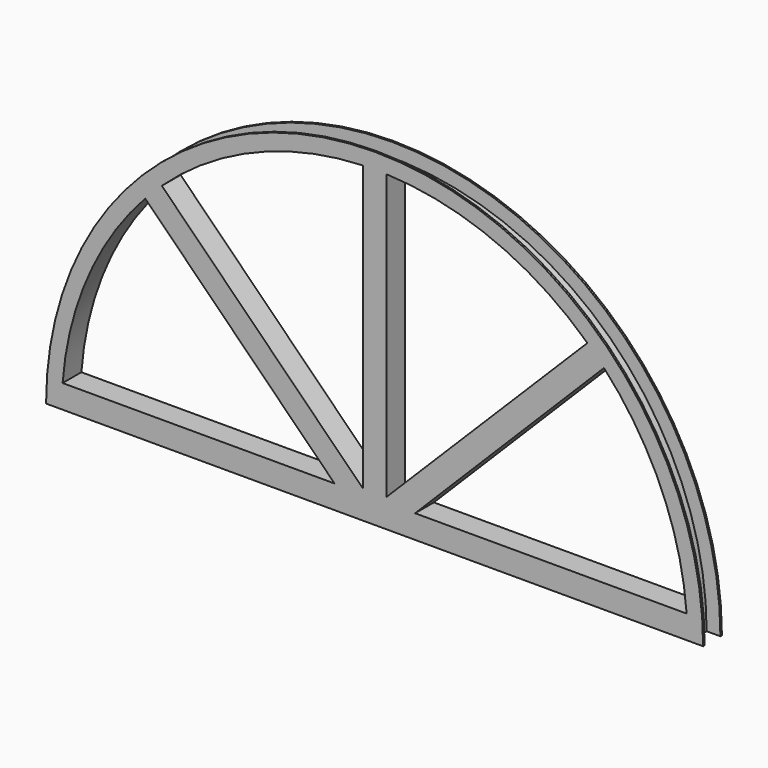
from build123d import *

# Parameters (mm, degrees)
F1_DEPTH     = 75
F2_T         = -6
F3_W         = 75
F3_H         = 75
F4_DEPTH     = 1000
F6_W         = 75
F6_H         = 75
F7_DEPTH     = 1000
F9_DEPTH     = 75
F11_DEPTH    = 75
F12_T        = 6
F12_T3_DEPTH = 87
F12_T6_ANGLE = 180.000000001
F12_T8_ANGLE = 180.000000001


# Not quite as in the source:
# - a shell that OpenCascade refuses in one call is made with other operations: the cavity is built on its own and cut out


with BuildPart() as f1:
    # F0 (on Front) → F1 (new body)
    with BuildSketch(Plane.XZ):
        with BuildLine():
            ThreePointArc((707.1067811865, 707.1067811865), (923.8795325113, 382.6834323651), (1000, 0))
            Line((1000, 0), (1050, 0))
            ThreePointArc((1050, 0), (0, 1050), (-1050, 0))
            Line((-1050, 0), (-1000, 0))
            ThreePointArc((-1000, 0), (-923.8795325113, 382.6834323651), (-707.1067811865, 707.1067811865))
            ThreePointArc((-707.1067811865, 707.1067811865), (-382.6834323651, 923.8795325113), (0, 1000))
            ThreePointArc((0, 1000), (382.6834323651, 923.8795325113), (707.1067811865, 707.1067811865))
        make_face()
    extrude(amount=F1_DEPTH)

    # F2
    f2_openings = [f1.faces().sort_by_distance(p)[0] for p in [
        (0, -37.5, 1050),
        (1025, -37.5, 0),
        (-1025, -37.5, 0),
    ]]
    offset(amount=F2_T, openings=f2_openings)

    # F3 (on Right) → F4 (join)
    with BuildSketch(Plane.YZ):
        with Locations((-37.5, 37.5)):
            Rectangle(F3_W, F3_H)
    extrude(amount=F4_DEPTH)

    # F5: F1 across plane


with BuildPart() as f1_1:
    add(f1.part)
    add(f1.part.mirror(Plane.YZ))

    # F6 (on face) → F7 (join)
    with BuildSketch(Plane(origin=(0, 0, 0), x_dir=(1, 0, 0), z_dir=(0, 0, -1))):
        with Locations((0, 37.5)):
            Rectangle(F6_W, F6_H)
    extrude(amount=-F7_DEPTH)

    # F8 (on face) → F9 (join)
    with BuildSketch(Plane.XZ):
        with BuildLine():
            Line((84.9014701911, 30.3333466038), (733.1259261111, 680.0929175221))
            ThreePointArc((733.1259261111, 680.0929175221), (707.1120975666, 707.1120975666), (680.0929175221, 733.1259261111))
            Line((680.0929175221, 733.1259261111), (-22.6996619852, 30.3333466038))
            Line((-22.6996619852, 30.3333466038), (84.9014701911, 30.3333466038))
        make_face()
        Polygon((-27.0138636644, 26.0191449246), (-22.6996619852, 30.3333466038), (-27.0138636644, 30.3333466038), align=None)
    extrude(amount=F9_DEPTH)

    # F10 (on Front) → F11 (join)
    with BuildSketch(Plane.XZ):
        Polygon((-97.2271824132, 44.1941738242), (-27.4779913529, 44.1941738242), (-30.0520382004, 83.0850467894), (-680.5902768921, 733.623285481), (-733.623285481, 680.5902768921), align=None)
    extrude(amount=F11_DEPTH)

    # F12: shell of thickness 6, made by hand


with BuildPart() as f12_core1:
    # F12_t2: copy of F1
    add(f1_1.part)

    # the walls: a layer under each face that stays
    f12_faces = [f12_core1.faces().sort_by_distance(p)[0] for p in [
        (0, 0, 525),
        (0, -37.5, 0),
        (0, -3, 1050),
        (-562.608271174, -37.5, 75),
        (-37.5, -37.5, 544.9148181113),
        (-382.6834323651, -37.5, 923.8795325113),
        (-916.5299048246, -37.5, 399.9661655218),
        (563.3230641949, -37.5, 75),
        (431.2942603709, -37.5, 377.5464587611),
        (916.5299048246, -37.5, 399.9661655218),
        (382.6834323651, -37.5, 923.8795325113),
        (37.5, -37.5, 544.9148181113),
        (358.7964587611, -37.5, 411.82946735),
        (-900, -6, 525),
        (0, -37.5, 1006),
        (-900, -69, 525),
        (0, -72, 1050),
        (0, -75, 525),
        (-430.57946735, -37.5, 377.5464587611),
        (-358.7964587611, -37.5, 411.82946735),
    ]]
    thicken(f12_faces, amount=-F12_T, mode=Mode.SUBTRACT)

    # F12_s4 → F12_t3 (cut)
    with BuildSketch(Plane.XZ.offset(-6)):
        Polygon((-128.0754349959, 75.0175735931), (-128.033008589, 69), (-113.5477272148, 69), (-123.7903679019, 79.2426406871), align=None)
        Polygon((-997.1237027469, 75.0555), (-997.183533759, 69), (-1003.6517512752, 69), (-1003.1666349615, 75.45), align=None)
        Polygon((-37.5175735931, 90.5754349959), (-31.5, 90.533008589), (-31.5, 76.0477272148), (-41.7426406871, 86.2903679019), align=None)
        Polygon((-37.55775, 999.236669836), (-31.5, 999.2966276337), (-31.5, 1005.5260092085), (-37.725, 1005.2924073995), align=None)
        Polygon((-680.0096855402, 733.1243649624), (-684.1734750272, 737.5246816678), (-688.7403961634, 733.2881233782), (-684.3355582092, 728.883285424), align=None)
        Polygon((-733.1243649624, 680.0096855402), (-737.5246816678, 684.1734750272), (-733.2881233782, 688.7403961634), (-728.883285424, 684.3355582092), align=None)
        Polygon((997.1237027469, 75.0555), (997.183533759, 69), (1003.6517512752, 69), (1003.1666349615, 75.45), align=None)
        Polygon((129.5050711853, 75.0176238001), (129.4625946308, 69), (115.0015064822, 69), (125.2149391782, 79.2376199873), align=None)
        Polygon((733.1244151101, 680.0097357472), (728.8782706586, 684.3305375094), (733.2831062303, 688.7458045437), (737.5246816678, 684.1734750272), align=None)
        Polygon((680.0096855402, 733.1243649624), (684.1734750272, 737.5246816678), (688.7403961634, 733.2881233782), (684.3355582092, 728.883285424), align=None)
        Polygon((37.55775, 999.236669836), (37.725, 1005.2924073995), (31.5, 1005.5260092085), (31.5, 999.2966276337), align=None)
        Polygon((37.5175735931, 90.5754349959), (31.5, 90.533008589), (31.5, 76.0477272148), (41.7426406871, 86.2903679019), align=None)
    extrude(amount=F12_T3_DEPTH, mode=Mode.SUBTRACT)

    # F12_s5 → F12_t6 (revolve, cut)
    with BuildSketch(Plane.XY):
        Polygon((-1006.06, -6.06), (-1006, 0), (-1000, 0), (-1000, -6), align=None)
    revolve(axis=Axis((0, -6, 0), (0, 1, 0)), revolution_arc=F12_T6_ANGLE, mode=Mode.SUBTRACT)

    # F12_s7 → F12_t8 (revolve, cut)
    with BuildSketch(Plane.XY):
        Polygon((-1006.06, -68.94), (-1000, -69), (-1000, -75), (-1006, -75), align=None)
    revolve(axis=Axis((0, -69, 0), (0, 1, 0)), revolution_arc=F12_T8_ANGLE, mode=Mode.SUBTRACT)


with BuildPart() as f1_2:
    add(f1_1.part)

    # what is left inside the walls is the cavity
    f12_cavity = [f12_core1.part.solids().sort_by_distance(p)[0] for p in [
        (0, -6.06, 337.333333),
    ]]
    add(f12_cavity, mode=Mode.SUBTRACT)


solid = f1_2.part
